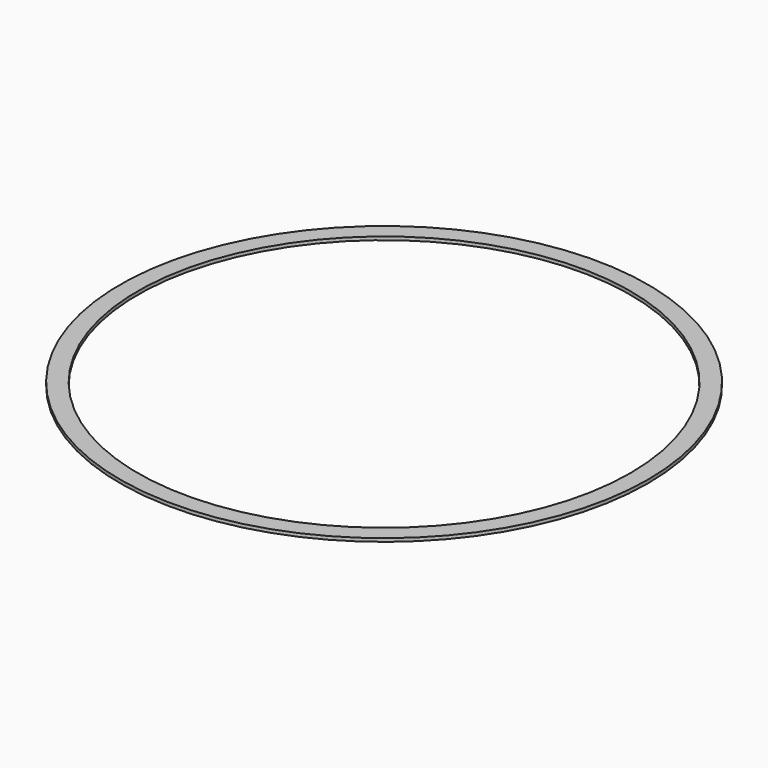
from build123d import *

# Parameters (mm, degrees)
F0_R     = 380.87173
F0_R_2   = 355.47173
F1_DEPTH = 4.7625


# Not quite as in the source:
# - a length typed as a fraction of an inch, garbled in the dataset ("3 / 203.2 mm" for 3/8 in), is restored


with BuildPart() as f1:
    # F0 (on Top) → F1 (new body)
    with BuildSketch(Plane.XY):
        Circle(F0_R)
        Circle(F0_R_2, mode=Mode.SUBTRACT)
    extrude(amount=F1_DEPTH)


solid = f1.part
